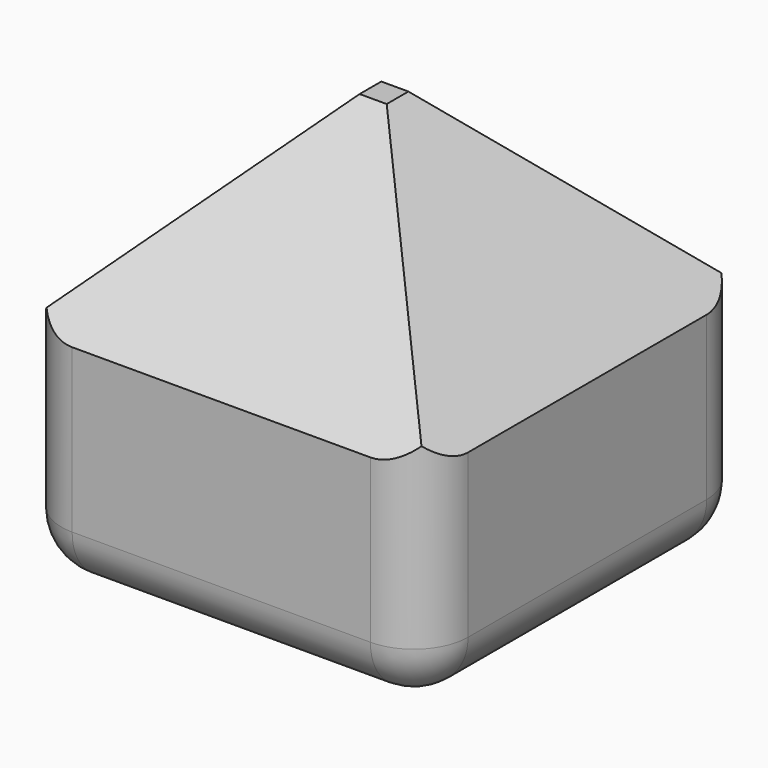
from build123d import *

# Parameters (mm, degrees)
F0_W         = 19.05
F0_H         = 19.05
F1_DEPTH     = 19.05
F2_SIZE      = 8.89
F3_T1_DEPTH  = 13.97
F3_T3_DEPTH  = 13.97
F3_T5_DEPTH  = 24.3105122421
F3_T7_DEPTH  = 13.97
F3_S11_W     = 2.54
F3_S11_H     = 2.54
F3_T12_DEPTH = 2.54
F3_S17_W     = 2.54
F3_S17_H     = 2.54
F3_T18_DEPTH = 2.54
F3_S23_W     = 2.54
F3_S23_H     = 2.54
F3_T24_DEPTH = 2.54
F3_S29_W     = 2.54
F3_S29_H     = 2.54
F3_T30_DEPTH = 2.54


# Not quite as in the source:
# - a fillet or chamfer that OpenCascade refuses, or shapes differently, is made with other operations: its cross-section is extruded or revolved along the edge and cut away or added


with BuildPart() as f1:
    # F0 (on Front) → F1 (new body)
    with BuildSketch(Plane.XZ):
        Rectangle(F0_W, F0_H)
    extrude(amount=F1_DEPTH)

    # F2
    f2_edges = [f1.edges().sort_by_distance(p)[0] for p in [
        (0, -19.05, 9.525),
        (0, 0, 9.525),
        (9.525, -9.525, 9.525),
        (-9.525, -9.525, 9.525),
    ]]
    chamfer(f2_edges, length=F2_SIZE)

    # F3: fillet of radius 2.54 on 9 edges, made by hand

    # F3_s2 → F3_t1 (cut)
    with BuildSketch(Plane.XY.offset(-6.985)):
        with BuildLine():
            ThreePointArc((9.525, -16.51), (8.7810512242, -18.3060512242), (6.985, -19.05))
            Line((6.985, -19.05), (9.525, -19.05))
            Line((9.525, -19.05), (9.525, -16.51))
        make_face()
        with BuildLine():
            ThreePointArc((-6.985, 0), (-8.7810512242, -0.7439487758), (-9.525, -2.54))
            Line((-9.525, -2.54), (-9.525, 0))
            Line((-9.525, 0), (-6.985, 0))
        make_face()
        with BuildLine():
            ThreePointArc((-6.985, -19.05), (-8.7810512242, -18.3060512242), (-9.525, -16.51))
            Line((-9.525, -16.51), (-9.525, -19.05))
            Line((-9.525, -19.05), (-6.985, -19.05))
        make_face()
        with BuildLine():
            ThreePointArc((9.525, -2.54), (8.7810512242, -0.7439487758), (6.985, 0))
            Line((6.985, 0), (9.525, 0))
            Line((9.525, 0), (9.525, -2.54))
        make_face()
    extrude(amount=F3_T1_DEPTH, mode=Mode.SUBTRACT)

    # F3_s4 → F3_t3 (cut)
    with BuildSketch(Plane.YZ.offset(-6.985)):
        with BuildLine():
            ThreePointArc((-16.51, -9.525), (-18.3060512242, -8.7810512242), (-19.05, -6.985))
            Line((-19.05, -6.985), (-19.05, -9.525))
            Line((-19.05, -9.525), (-16.51, -9.525))
        make_face()
        with BuildLine():
            ThreePointArc((0, -6.985), (-0.7439487758, -8.7810512242), (-2.54, -9.525))
            Line((-2.54, -9.525), (0, -9.525))
            Line((0, -9.525), (0, -6.985))
        make_face()
    extrude(amount=F3_T3_DEPTH, mode=Mode.SUBTRACT)

    # F3_s6 → F3_t5 (cut)
    with BuildSketch(Plane.XZ.offset(-2.6302561211)):
        with BuildLine():
            ThreePointArc((-9.525, -0.4171024484), (-9.3316540126, 0.5549134698), (-8.7810512242, 1.3789487758))
            Line((-8.7810512242, 1.3789487758), (-9.525, 0.635))
            Line((-9.525, 0.635), (-9.525, -0.4171024484))
        make_face()
    extrude(amount=F3_T5_DEPTH, mode=Mode.SUBTRACT)

    # F3_s8 → F3_t7 (cut)
    with BuildSketch(Plane.XZ.offset(2.54)):
        with BuildLine():
            ThreePointArc((-6.985, -9.525), (-8.7810512242, -8.7810512242), (-9.525, -6.985))
            Line((-9.525, -6.985), (-9.525, -9.525))
            Line((-9.525, -9.525), (-6.985, -9.525))
        make_face()
        with BuildLine():
            ThreePointArc((9.525, -6.985), (8.7810512242, -8.7810512242), (6.985, -9.525))
            Line((6.985, -9.525), (9.525, -9.525))
            Line((9.525, -9.525), (9.525, -6.985))
        make_face()
    extrude(amount=F3_T7_DEPTH, mode=Mode.SUBTRACT)


with BuildPart() as f3_tool10:
    # F3_s11 → F3_t12 (new body)
    with BuildSketch(Plane.YZ.offset(6.985)):
        with Locations((-17.78, -8.255)):
            Rectangle(F3_S11_W, F3_S11_H)
    extrude(amount=F3_T12_DEPTH)

    # F3_s13 → F3_t14 (revolve, cut)
    with BuildSketch(Plane(origin=(6.985, -16.51, -6.985), x_dir=(0, 0.7071067812, 0.7071067812), z_dir=(0, 0.7071067812, -0.7071067812))):
        with BuildLine():
            ThreePointArc((0, -2.54), (2.54, 0), (0, 2.54))
            Line((0, 2.54), (0, -2.54))
        make_face()
    revolve(axis=Axis((6.985, -16.51, -6.985), (1, 0, 0)), mode=Mode.SUBTRACT)


with BuildPart() as f1_1:
    add(f1.part)

    # F3_t9: cut F3_tool10
    add(f3_tool10.part, mode=Mode.SUBTRACT)


with BuildPart() as f3_tool16:
    # F3_s17 → F3_t18 (new body)
    with BuildSketch(Plane.XY.offset(-6.985)):
        with Locations((-8.255, -17.78)):
            Rectangle(F3_S17_W, F3_S17_H)
    extrude(amount=-F3_T18_DEPTH)

    # F3_s19 → F3_t20 (revolve, cut)
    with BuildSketch(Plane(origin=(-6.985, -16.51, -6.985), x_dir=(0.7071067812, 0.7071067812, 0), z_dir=(-0.7071067812, 0.7071067812, 0))):
        with BuildLine():
            ThreePointArc((0, -2.54), (2.54, 0), (0, 2.54))
            Line((0, 2.54), (0, -2.54))
        make_face()
    revolve(axis=Axis((-6.985, -16.51, -6.985), (0, 0, -1)), mode=Mode.SUBTRACT)


with BuildPart() as f1_2:
    add(f1_1.part)

    # F3_t15: cut F3_tool16
    add(f3_tool16.part, mode=Mode.SUBTRACT)


with BuildPart() as f3_tool22:
    # F3_s23 → F3_t24 (new body)
    with BuildSketch(Plane.XZ.offset(2.54)):
        with Locations((-8.255, -8.255)):
            Rectangle(F3_S23_W, F3_S23_H)
    extrude(amount=-F3_T24_DEPTH)

    # F3_s25 → F3_t26 (revolve, cut)
    with BuildSketch(Plane(origin=(-6.985, -2.54, -6.985), x_dir=(0.7071067812, 0, 0.7071067812), z_dir=(-0.7071067812, 0, 0.7071067812))):
        with BuildLine():
            ThreePointArc((0, -2.54), (2.54, 0), (0, 2.54))
            Line((0, 2.54), (0, -2.54))
        make_face()
    revolve(axis=Axis((-6.985, -2.54, -6.985), (0, 1, 0)), mode=Mode.SUBTRACT)


with BuildPart() as f1_3:
    add(f1_2.part)

    # F3_t21: cut F3_tool22
    add(f3_tool22.part, mode=Mode.SUBTRACT)


with BuildPart() as f3_tool28:
    # F3_s29 → F3_t30 (new body)
    with BuildSketch(Plane.YZ.offset(6.985)):
        with Locations((-1.27, -8.255)):
            Rectangle(F3_S29_W, F3_S29_H)
    extrude(amount=F3_T30_DEPTH)

    # F3_s31 → F3_t32 (revolve, cut)
    with BuildSketch(Plane(origin=(6.985, -2.54, -6.985), x_dir=(0, -0.7071067812, 0.7071067812), z_dir=(0, 0.7071067812, 0.7071067812))):
        with BuildLine():
            ThreePointArc((0, -2.54), (2.54, 0), (0, 2.54))
            Line((0, 2.54), (0, -2.54))
        make_face()
    revolve(axis=Axis((6.985, -2.54, -6.985), (1, 0, 0)), mode=Mode.SUBTRACT)


with BuildPart() as f1_4:
    add(f1_3.part)

    # F3_t27: cut F3_tool28
    add(f3_tool28.part, mode=Mode.SUBTRACT)


solid = f1_4.part
